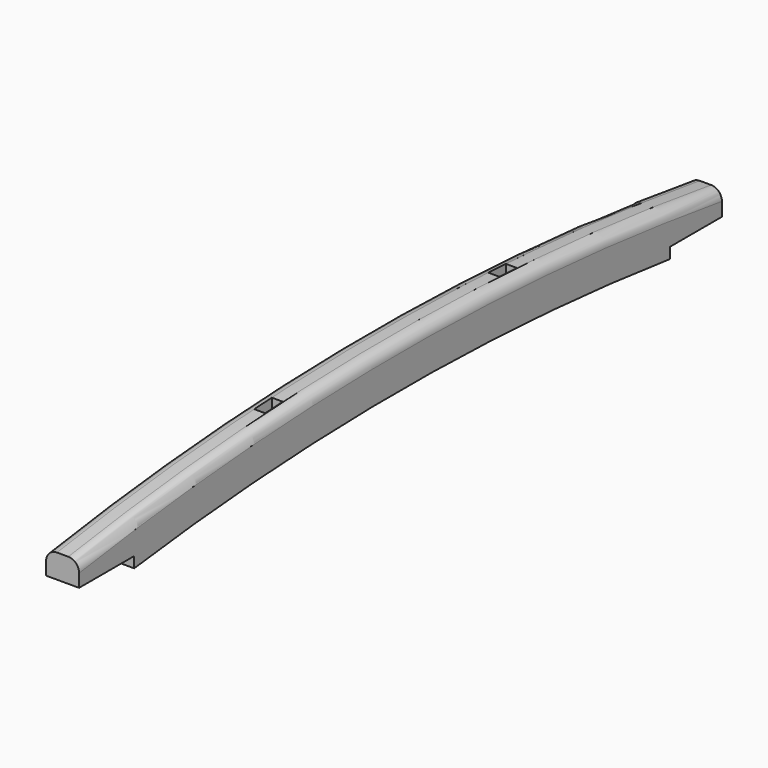
from build123d import *

# Parameters (mm, degrees)
F1_DEPTH = 152.4
F2_R     = 50
F4_W     = 50.8
F4_H     = 101.6
F5_DEPTH = 152.4


with BuildPart() as f1:
    # F0 (on Right) → F1 (new body)
    with BuildSketch(Plane.YZ):
        with BuildLine():
            ThreePointArc((-1546.8, -50), (0, 49.0106103665), (1546.8, -50))
            Line((1546.8, -50), (1546.8, 0))
            Line((1546.8, 0), (1846.1961399702, 0))
            Line((1846.1961399702, 0), (1846.1961399702, 113.2689997187))
            ThreePointArc((1846.1961399702, 113.2689997187), (-9.4967662084, 252.2069546258), (-1864.9735382658, 110.4118005804))
            Line((-1864.9735382658, 110.4118005804), (-1864.9735382658, 0))
            Line((-1864.9735382658, 0), (-1546.8, 0))
            Line((-1546.8, 0), (-1546.8, -50))
        make_face()
    extrude(amount=F1_DEPTH)

    # F2
    f2_edges = [f1.edges().sort_by_distance(p)[0] for p in [
        (152.4, -9.496766, 252.206955),
        (0, -9.496766, 252.206955),
    ]]
    fillet(f2_edges, radius=F2_R)

    # F4 (on face) → F5 (cut)
    with BuildSketch(Plane(origin=(0, -0.086110522, 111.8475621363), x_dir=(1, 0, 0), z_dir=(0, -0.0007698916, 0.9999997036))):
        with Locations((76.2, -675.8)):
            Rectangle(F4_W, F4_H)
        with Locations((76.2, 675.8)):
            Rectangle(F4_W, F4_H)
    extrude(amount=F5_DEPTH, mode=Mode.SUBTRACT)


solid = f1.part
